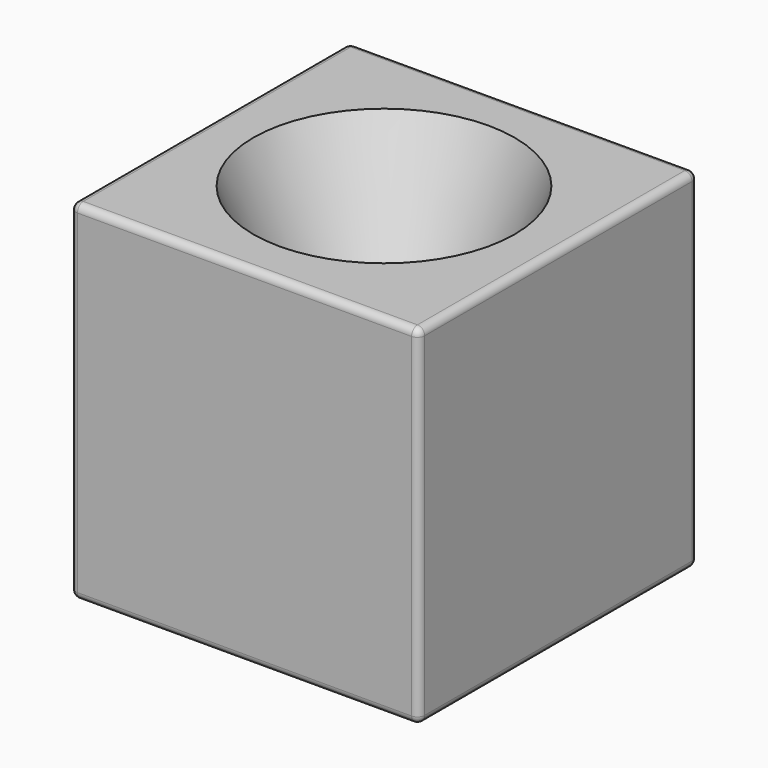
from build123d import *

# Parameters (mm, degrees)
F0_W           = 48
F0_H           = 48
F1_DEPTH       = 48
F2_R           = 1
F3_R           = 1
F4_T1_DEPTH    = 46
F4_T3_DEPTH    = 46
F4_T5_DEPTH    = 46
F4_S9_W        = 1
F4_S9_H        = 1
F4_T10_DEPTH   = 1
F4_S15_W       = 1
F4_S15_H       = 1
F4_T16_DEPTH   = 1
F4_S21_W       = 1
F4_S21_H       = 1
F4_T22_DEPTH   = 1
F4_S27_W       = 1
F4_S27_H       = 1
F4_T28_DEPTH   = 1
F4_T32_ANGLE   = 90
F4_T34_ANGLE   = 90
F6_D           = 18
F6_CSINK_D     = 36
F6_CSINK_ANGLE = 45


# Not quite as in the source:
# - a fillet or chamfer that OpenCascade refuses, or shapes differently, is made with other operations: its cross-section is extruded or revolved along the edge and cut away or added


with BuildPart() as f1:
    # F0 (on Front) → F1 (new body)
    with BuildSketch(Plane.XZ):
        Rectangle(F0_W, F0_H)
    extrude(amount=F1_DEPTH)

    # F2
    f2_edges = [f1.edges().sort_by_distance(p)[0] for p in [
        (24, -24, 24),
    ]]
    fillet(f2_edges, radius=F2_R)

    # F3
    f3_edges = [f1.edges().sort_by_distance(p)[0] for p in [
        (-24, -24, 24),
        (-0.5, 0, 24),
        (-0.5, -48, 24),
    ]]
    fillet(f3_edges, radius=F3_R)

    # F4: fillet of radius 1 on 8 edges, made by hand

    # F4_s2 → F4_t1 (cut)
    with BuildSketch(Plane.XY.offset(-23)):
        with BuildLine():
            ThreePointArc((-23, -48), (-23.7071067812, -47.7071067812), (-24, -47))
            Line((-24, -47), (-24, -48))
            Line((-24, -48), (-23, -48))
        make_face()
        with BuildLine():
            ThreePointArc((-23, 0), (-23.7071067812, -0.2928932188), (-24, -1))
            Line((-24, -1), (-24, 0))
            Line((-24, 0), (-23, 0))
        make_face()
    extrude(amount=F4_T1_DEPTH, mode=Mode.SUBTRACT)

    # F4_s4 → F4_t3 (cut)
    with BuildSketch(Plane.YZ.offset(-23)):
        with BuildLine():
            ThreePointArc((0, -23), (-0.2928932188, -23.7071067812), (-1, -24))
            Line((-1, -24), (0, -24))
            Line((0, -24), (0, -23))
        make_face()
        with BuildLine():
            ThreePointArc((-48, -23), (-47.7071067812, -23.7071067812), (-47, -24))
            Line((-47, -24), (-48, -24))
            Line((-48, -24), (-48, -23))
        make_face()
    extrude(amount=F4_T3_DEPTH, mode=Mode.SUBTRACT)

    # F4_s6 → F4_t5 (cut)
    with BuildSketch(Plane.XZ.offset(1)):
        with BuildLine():
            ThreePointArc((-24, -23), (-23.7071067812, -23.7071067812), (-23, -24))
            Line((-23, -24), (-24, -24))
            Line((-24, -24), (-24, -23))
        make_face()
        with BuildLine():
            ThreePointArc((24, -23), (23.7071067812, -23.7071067812), (23, -24))
            Line((23, -24), (24, -24))
            Line((24, -24), (24, -23))
        make_face()
    extrude(amount=F4_T5_DEPTH, mode=Mode.SUBTRACT)


with BuildPart() as f4_tool8:
    # F4_s9 → F4_t10 (new body)
    with BuildSketch(Plane.XZ.offset(1)):
        with Locations((-23.5, 23.5)):
            Rectangle(F4_S9_W, F4_S9_H)
    extrude(amount=-F4_T10_DEPTH)

    # F4_s11 → F4_t12 (revolve, cut)
    with BuildSketch(Plane(origin=(-23, -1, 23), x_dir=(0.7071067812, 0, -0.7071067812), z_dir=(0.7071067812, 0, 0.7071067812))):
        with BuildLine():
            ThreePointArc((0, -1), (1, 0), (0, 1))
            Line((0, 1), (0, -1))
        make_face()
    revolve(axis=Axis((-23, -1, 23), (0, 1, 0)), mode=Mode.SUBTRACT)


with BuildPart() as f1_1:
    add(f1.part)

    # F4_t7: cut F4_tool8
    add(f4_tool8.part, mode=Mode.SUBTRACT)


with BuildPart() as f4_tool14:
    # F4_s15 → F4_t16 (new body)
    with BuildSketch(Plane.XZ.offset(47)):
        with Locations((-23.5, 23.5)):
            Rectangle(F4_S15_W, F4_S15_H)
    extrude(amount=F4_T16_DEPTH)

    # F4_s17 → F4_t18 (revolve, cut)
    with BuildSketch(Plane(origin=(-23, -47, 23), x_dir=(0.7071067812, 0, -0.7071067812), z_dir=(-0.7071067812, 0, -0.7071067812))):
        with BuildLine():
            ThreePointArc((0, -1), (1, 0), (0, 1))
            Line((0, 1), (0, -1))
        make_face()
    revolve(axis=Axis((-23, -47, 23), (0, -1, 0)), mode=Mode.SUBTRACT)


with BuildPart() as f1_2:
    add(f1_1.part)

    # F4_t13: cut F4_tool14
    add(f4_tool14.part, mode=Mode.SUBTRACT)


with BuildPart() as f4_tool20:
    # F4_s21 → F4_t22 (new body)
    with BuildSketch(Plane.XZ.offset(47)):
        with Locations((-23.5, -23.5)):
            Rectangle(F4_S21_W, F4_S21_H)
    extrude(amount=F4_T22_DEPTH)

    # F4_s23 → F4_t24 (revolve, cut)
    with BuildSketch(Plane(origin=(-23, -47, -23), x_dir=(0.7071067812, 0, 0.7071067812), z_dir=(0.7071067812, 0, -0.7071067812))):
        with BuildLine():
            ThreePointArc((0, -1), (1, 0), (0, 1))
            Line((0, 1), (0, -1))
        make_face()
    revolve(axis=Axis((-23, -47, -23), (0, -1, 0)), mode=Mode.SUBTRACT)


with BuildPart() as f1_3:
    add(f1_2.part)

    # F4_t19: cut F4_tool20
    add(f4_tool20.part, mode=Mode.SUBTRACT)


with BuildPart() as f4_tool26:
    # F4_s27 → F4_t28 (new body)
    with BuildSketch(Plane.XZ.offset(1)):
        with Locations((-23.5, -23.5)):
            Rectangle(F4_S27_W, F4_S27_H)
    extrude(amount=-F4_T28_DEPTH)

    # F4_s29 → F4_t30 (revolve, cut)
    with BuildSketch(Plane(origin=(-23, -1, -23), x_dir=(0.7071067812, 0, 0.7071067812), z_dir=(-0.7071067812, 0, 0.7071067812))):
        with BuildLine():
            ThreePointArc((0, -1), (1, 0), (0, 1))
            Line((0, 1), (0, -1))
        make_face()
    revolve(axis=Axis((-23, -1, -23), (0, 1, 0)), mode=Mode.SUBTRACT)


with BuildPart() as f1_4:
    add(f1_3.part)

    # F4_t25: cut F4_tool26
    add(f4_tool26.part, mode=Mode.SUBTRACT)

    # F4_s31 → F4_t32 (revolve, cut)
    with BuildSketch(Plane.XZ.offset(1)):
        with BuildLine():
            ThreePointArc((24, -23), (23.7071067812, -23.7071067812), (23, -24))
            Line((23, -24), (24, -24))
            Line((24, -24), (24, -23))
        make_face()
    revolve(axis=Axis((23, -1, -24), (0, 0, 1)), revolution_arc=F4_T32_ANGLE, mode=Mode.SUBTRACT)

    # F4_s33 → F4_t34 (revolve, cut)
    with BuildSketch(Plane.XZ.offset(47)):
        with BuildLine():
            ThreePointArc((24, -23), (23.7071067812, -23.7071067812), (23, -24))
            Line((23, -24), (24, -24))
            Line((24, -24), (24, -23))
        make_face()
    revolve(axis=Axis((23, -47, -24), (0, 0, -1)), revolution_arc=F4_T34_ANGLE, mode=Mode.SUBTRACT)

    # F6 (through all)
    with Locations(Plane.XY.offset(24)):
        with Locations((0, -24)):
            CounterSinkHole(F6_D / 2, F6_CSINK_D / 2, counter_sink_angle=F6_CSINK_ANGLE)


solid = f1_4.part
